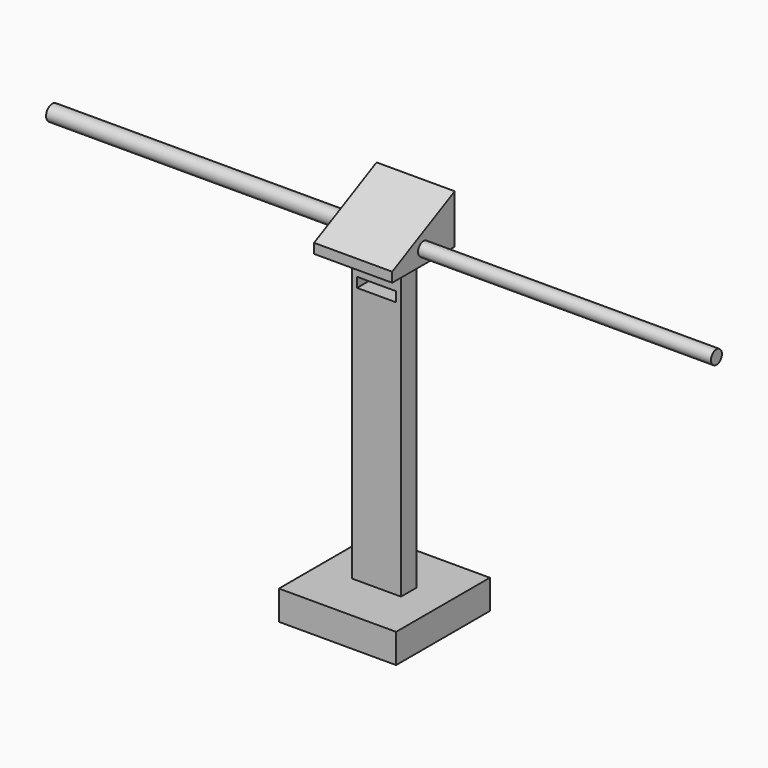
from build123d import *

# Parameters (mm, degrees)
F0_W      = 60
F0_H      = 60
F1_DEPTH  = 15
F2_W      = 25
F2_H      = 10
F3_DEPTH  = 150
F4_W      = 40
F4_H      = 40
F4_W_2    = 25
F4_H_2    = 10
F5_DEPTH  = 25
F6_SIZE2  = 39.99999
F6_SIZE   = 19.99999
F7_W      = 20
F7_H      = 5
F8_DEPTH  = 25
F9_R      = 3.5
F10_DEPTH = 150
F11_R     = 4
F12_DEPTH = 150


# Not quite as in the source:
# - a fillet or chamfer is up to 0.001 mm smaller than in the source, because OpenCascade refuses the exact size


with BuildPart() as f1:
    # F0 (on Top) → F1 (new body)
    with BuildSketch(Plane.XY):
        Rectangle(F0_W, F0_H)
    extrude(amount=F1_DEPTH)

    # F2 (on face) → F3 (join)
    with BuildSketch(Plane.XY.offset(15)):
        Rectangle(F2_W, F2_H)
    extrude(amount=F3_DEPTH)

    # F4 (on face) → F5 (join)
    with BuildSketch(Plane.XY.offset(165)):
        Rectangle(F4_W, F4_H)
        Rectangle(F4_W_2, F4_H_2, mode=Mode.SUBTRACT)
        Rectangle(F4_W_2, F4_H_2)
    extrude(amount=F5_DEPTH)

    # F6 (size 20 and 40 in the source; OpenCascade refuses exactly that, so slightly less here)
    f6_edges = [f1.edges().sort_by_distance(p)[0] for p in [
        (0, -20, 190),
    ]]
    f6_side = f1.faces().sort_by_distance((0, -20, 177.5))[0]
    chamfer(f6_edges, length=F6_SIZE, length2=F6_SIZE2, reference=f6_side)

    # F7 (on face) → F8 (cut)
    with BuildSketch(Plane.XZ.offset(5)):
        with Locations((0, 149.3448019028)):
            Rectangle(F7_W, F7_H)
    extrude(amount=-F8_DEPTH, mode=Mode.SUBTRACT)

    # F9 (on face) → F10 (join)
    with BuildSketch(Plane.YZ.offset(20)):
        with Locations((0, 172.1751581079)):
            Circle(F9_R)
    extrude(amount=F10_DEPTH)

    # F11 (on face) → F12 (join)
    with BuildSketch(Plane(origin=(-20, 0, 0), x_dir=(0, -1, 0), z_dir=(-1, 0, 0))):
        with Locations((0, 171.8452831515)):
            Circle(F11_R)
    extrude(amount=F12_DEPTH)


solid = f1.part
